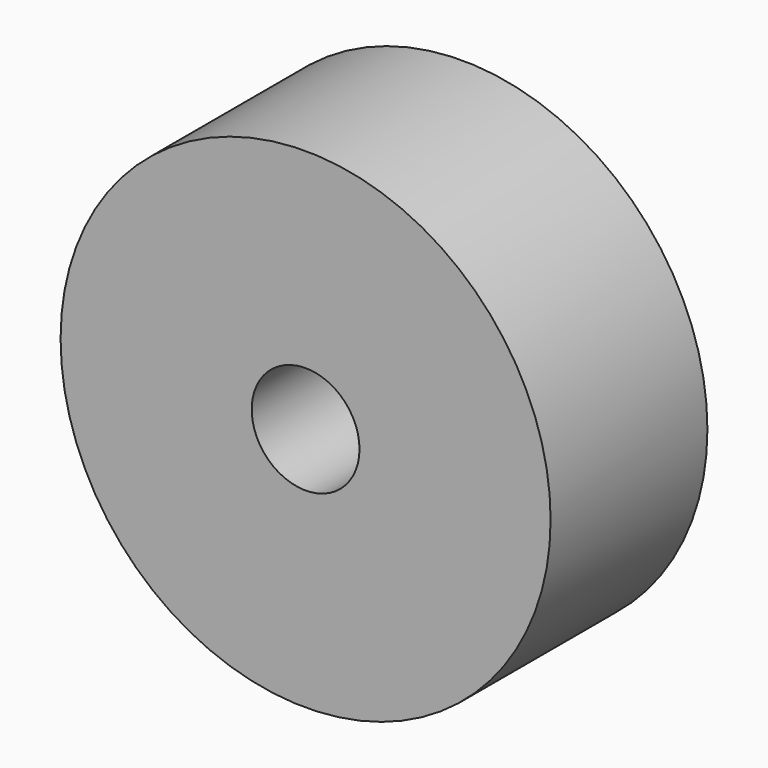
from build123d import *

# Parameters (mm, degrees)
F0_R     = 31.75
F0_R_2   = 6.985
F1_DEPTH = 25.4


# Not quite as in the source:
# - a feature names something its author has since deleted; it is built from what else it names


with BuildPart() as f1:
    # F0 (on Front) → F1 (new body)
    with BuildSketch(Plane.XZ):
        Circle(F0_R)
        Circle(F0_R_2, mode=Mode.SUBTRACT)
    extrude(amount=F1_DEPTH)


solid = f1.part
